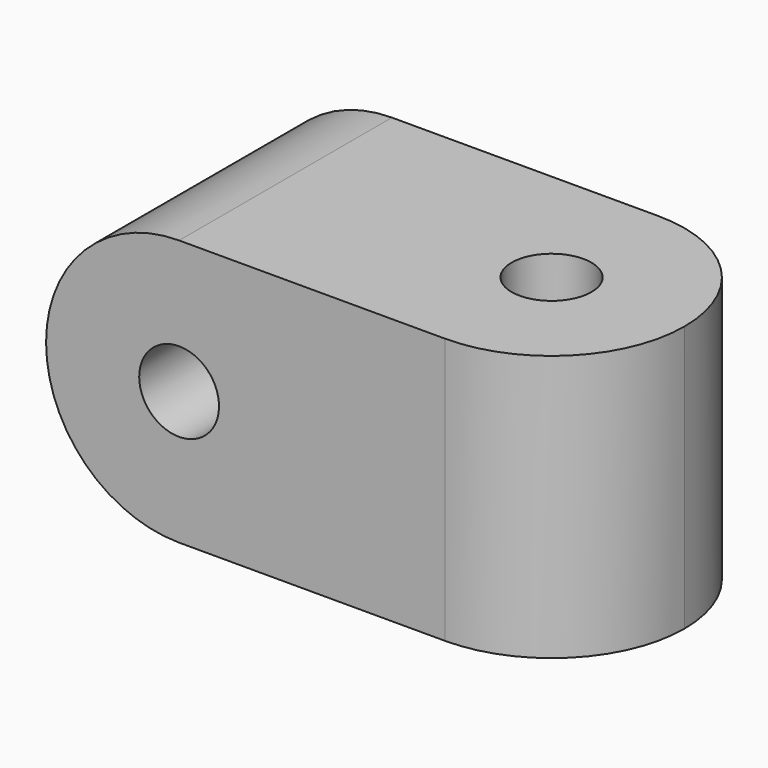
from build123d import *

# Parameters (mm, degrees)
F0_W     = 39.9999970493
F0_H     = 20
F1_DEPTH = 20
F3_D     = 6
F5_D     = 6
F6_R     = 9.99999
F7_R     = 9.99999


# Not quite as in the source:
# - a fillet or chamfer is up to 0.001 mm smaller than in the source, because OpenCascade refuses the exact size


with BuildPart() as f1:
    # F0 (on Top) → F1 (new body)
    with BuildSketch(Plane.XY):
        with Locations((19.9999985246, 10)):
            Rectangle(F0_W, F0_H)
    extrude(amount=F1_DEPTH)

    # F3 (through all)
    with Locations(Plane.XY.offset(20)):
        with Locations((30.0000011921, 10)):
            Hole(F3_D / 2)

    # F5 (through all)
    with Locations(Plane.XZ):
        with Locations((10, 10)):
            Hole(F5_D / 2)

    # F6 (radius 10 in the source; OpenCascade refuses exactly that, so slightly less here)
    f6_edges = [f1.edges().sort_by_distance(p)[0] for p in [
        (39.999997, 0, 10),
        (39.999997, 20, 10),
    ]]
    fillet(f6_edges, radius=F6_R)

    # F7 (radius 10 in the source; OpenCascade refuses exactly that, so slightly less here)
    f7_edges = [f1.edges().sort_by_distance(p)[0] for p in [
        (0, 10, 0),
        (0, 10, 20),
    ]]
    fillet(f7_edges, radius=F7_R)


solid = f1.part
